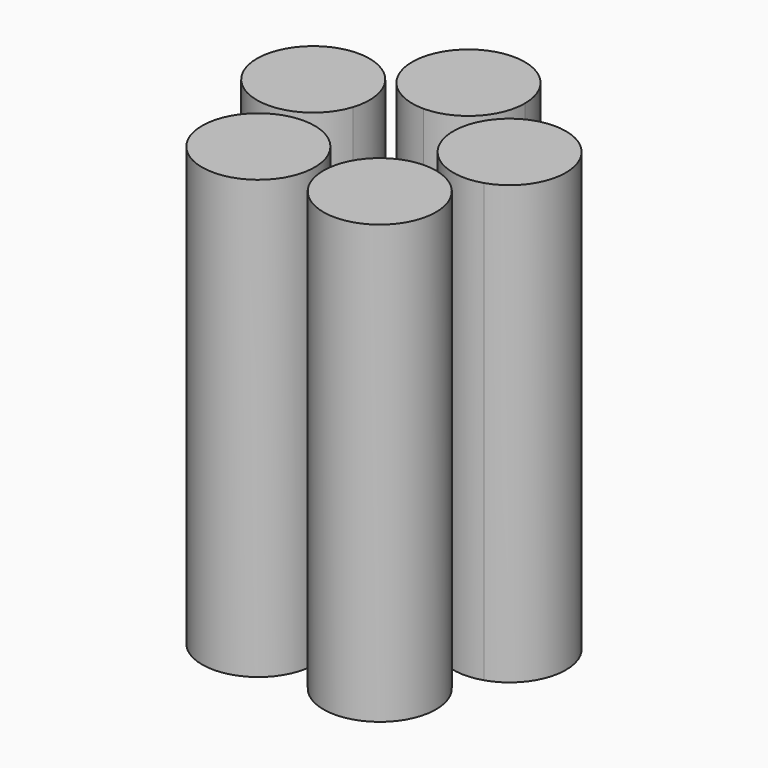
from build123d import *

# Parameters (mm, degrees)
F1_DEPTH        = 70
F1_COPIES_COUNT = 5


# Not quite as in the source:
# - a pattern or mirror of a feature is missing from the dataset's text; its kind, count and spacing are read off the source's solid


with BuildPart() as f1:
    # F0 (on Top) → F1 (new body)
    with BuildSketch(Plane.XY):
        with BuildLine():
            ThreePointArc((0, 7.51), (6.3639610307, 10.1460389693), (9, 16.51))
            ThreePointArc((9, 16.51), (-6.3639610307, 22.8739610307), (0, 7.51))
        make_face()
    extrude(amount=F1_DEPTH)


with BuildPart() as f1_copies_1:
    # F1_copies: instance of F1
    add(f1.part.rotate(Axis((0, 0, 0), (0, 0, 1)), 1 * 360 / F1_COPIES_COUNT))


with BuildPart() as f1_copies_2:
    # F1_copies: instance of F1
    add(f1.part.rotate(Axis((0, 0, 0), (0, 0, 1)), 2 * 360 / F1_COPIES_COUNT))


with BuildPart() as f1_copies_3:
    # F1_copies: instance of F1
    add(f1.part.rotate(Axis((0, 0, 0), (0, 0, 1)), 3 * 360 / F1_COPIES_COUNT))


with BuildPart() as f1_copies_4:
    # F1_copies: instance of F1
    add(f1.part.rotate(Axis((0, 0, 0), (0, 0, 1)), 4 * 360 / F1_COPIES_COUNT))


solid = Compound([f1.part, f1_copies_1.part, f1_copies_2.part, f1_copies_3.part, f1_copies_4.part])
